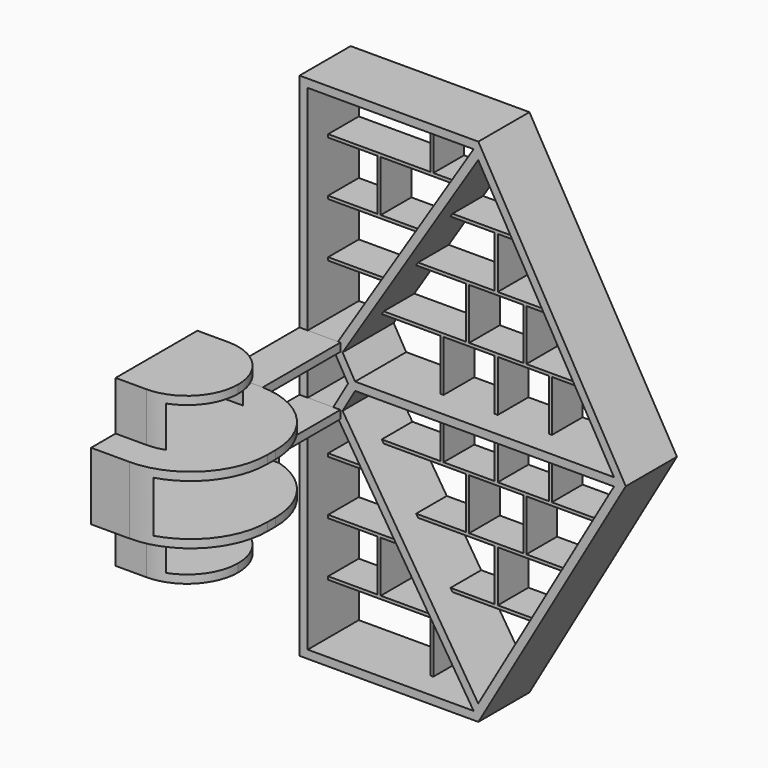
from build123d import *

# Parameters (mm, degrees)
F2_DEPTH    = 125
F1_W        = 6
F1_H        = 100
F3_DEPTH    = 75
F4_W        = 6
F4_H        = 80
F5_DEPTH    = 160
F4_H_2      = 100
F6_DEPTH    = 80
F7_R        = 99.99999
F7_2_R      = 99.99999
F8_DEPTH    = 225
F9_T1_DEPTH = 882


# Not quite as in the source:
# - a fillet or chamfer that OpenCascade refuses, or shapes differently, is made with other operations: its cross-section is extruded or revolved along the edge and cut away or added
# - a fillet or chamfer is up to 0.001 mm smaller than in the source, because OpenCascade refuses the exact size
# - a feature names something its author has since deleted; it is built from what else it names


with BuildPart() as f2:
    # F1 (on Front) → F2 (new body)
    with BuildSketch(Plane.XZ):
        Polygon((0, 1000), (0, 0), (350, 0), (638.6751345948, 500), (350, 1000), align=None)
        Polygon((16, 884), (16, 984), (216, 984), (222, 984), (340.762395693, 984), (349.7876249334, 968.3678444056), (431.9837382249, 826), (435.4478398401, 820), (493.182866759, 720), (496.6469683742, 714), (554.3819952931, 614), (557.8460969083, 608), (615.5811238272, 508), (620.1999259807, 500), (615.5811238272, 492), (557.8460969083, 392), (554.3819952931, 386), (496.6469683742, 286), (493.182866759, 280), (435.4478398401, 180), (431.9837382249, 174), (349.7876249334, 31.6321555944), (340.762395693, 16), (222, 16), (216, 16), (16, 16), (16, 116), (16, 122), (16, 222), (16, 228), (16, 328), (16, 334), (16, 434), (16, 450), (16, 550), (16, 566), (16, 666), (16, 672), (16, 772), (16, 778), (16, 878), align=None, mode=Mode.SUBTRACT)
        Polygon((236.0177204531, 508), (108.72391992, 508), (113.3427220735, 500), (108.72391992, 492), (236.0177204531, 492), (242.0177204531, 492), (342.0177204531, 492), (348.0177204531, 492), (448.0177204531, 492), (454.0177204531, 492), (615.5811238272, 492), (620.1999259807, 500), (615.5811238272, 508), (454.0177204531, 508), (448.0177204531, 508), (348.0177204531, 508), (342.0177204531, 508), (242.0177204531, 508), align=None)
        Polygon((84.2628335475, 449.6321555944), (75.237604307, 434), (138.7602816721, 334), (142.571642314, 328), (206.094319679, 228), (209.905680321, 222), (273.428357686, 122), (277.2397183279, 116), (340.762395693, 16), (349.7876249334, 31.6321555944), (259.3517584601, 174), (255.5403978182, 180), (192.0177204531, 280), (188.2063598112, 286), (124.6836824461, 386), (120.8723218042, 392), align=None)
        Polygon((349.7876249334, 968.3678444056), (340.762395693, 984), (277.2397183279, 884), (273.428357686, 878), (209.905680321, 778), (206.094319679, 772), (142.571642314, 672), (138.7602816721, 666), (75.237604307, 566), (84.2628335475, 550.3678444056), (120.8723218042, 608), (124.6836824461, 614), (188.2063598112, 714), (192.0177204531, 720), (255.5403978182, 820), (259.3517584601, 826), align=None)
        Polygon((75.237604307, 566), (16, 566), (16, 550), (66, 550), (94.8675134595, 500), (66, 450), (16, 450), (16, 434), (75.237604307, 434), (84.2628335475, 449.6321555944), (108.72391992, 492), (113.3427220735, 500), (108.72391992, 508), (84.2628335475, 550.3678444056), align=None)
    extrude(amount=F2_DEPTH)

    # F1 (on Front) → F3 (join)
    with BuildSketch(Plane.XZ):
        Polygon((112.9528401605, 122), (16, 122), (16, 116), (216, 116), (222, 116), (277.2397183279, 116), (273.428357686, 122), (118.9528401605, 122), align=None)
        with Locations((219, 66)):
            Rectangle(F1_W, F1_H)
        with Locations((115.9528401605, 172)):
            Rectangle(F1_W, F1_H)
        Polygon((206.094319679, 228), (16, 228), (16, 222), (112.9528401605, 222), (118.9528401605, 222), (209.905680321, 222), align=None)
        Polygon((138.7602816721, 334), (16, 334), (16, 328), (142.571642314, 328), align=None)
        Polygon((342.0177204531, 180), (255.5403978182, 180), (259.3517584601, 174), (431.9837382249, 174), (435.4478398401, 180), (348.0177204531, 180), align=None)
        with Locations((345.0177204531, 230)):
            Rectangle(F1_W, F1_H)
        Polygon((286.0177204531, 286), (188.2063598112, 286), (192.0177204531, 280), (342.0177204531, 280), (348.0177204531, 280), (493.182866759, 280), (496.6469683742, 286), (404.0177204531, 286), (398.0177204531, 286), (292.0177204531, 286), align=None)
        with Locations((289.0177204531, 336)):
            Rectangle(F1_W, F1_H)
        with Locations((401.0177204531, 336)):
            Rectangle(F1_W, F1_H)
        Polygon((236.0177204531, 392), (120.8723218042, 392), (124.6836824461, 386), (286.0177204531, 386), (292.0177204531, 386), (398.0177204531, 386), (404.0177204531, 386), (554.3819952931, 386), (557.8460969083, 392), (454.0177204531, 392), (448.0177204531, 392), (348.0177204531, 392), (342.0177204531, 392), (242.0177204531, 392), align=None)
        with Locations((345.0177204531, 442)):
            Rectangle(F1_W, F1_H)
        with Locations((239.0177204531, 442)):
            Rectangle(F1_W, F1_H)
        with Locations((451.0177204531, 442)):
            Rectangle(F1_W, F1_H)
        with Locations((401.0177204531, 664)):
            Rectangle(F1_W, F1_H)
        Polygon((496.6469683742, 714), (493.182866759, 720), (348.0177204531, 720), (342.0177204531, 720), (192.0177204531, 720), (188.2063598112, 714), (286.0177204531, 714), (292.0177204531, 714), (398.0177204531, 714), (404.0177204531, 714), align=None)
        with Locations((345.0177204531, 770)):
            Rectangle(F1_W, F1_H)
        Polygon((557.8460969083, 608), (554.3819952931, 614), (404.0177204531, 614), (398.0177204531, 614), (292.0177204531, 614), (286.0177204531, 614), (124.6836824461, 614), (120.8723218042, 608), (236.0177204531, 608), (242.0177204531, 608), (342.0177204531, 608), (348.0177204531, 608), (448.0177204531, 608), (454.0177204531, 608), align=None)
        with Locations((451.0177204531, 558)):
            Rectangle(F1_W, F1_H)
        with Locations((239.0177204531, 558)):
            Rectangle(F1_W, F1_H)
        with Locations((345.0177204531, 558)):
            Rectangle(F1_W, F1_H)
        Polygon((142.571642314, 672), (16, 672), (16, 666), (138.7602816721, 666), align=None)
        Polygon((112.9528401605, 778), (16, 778), (16, 772), (206.094319679, 772), (209.905680321, 778), (118.9528401605, 778), align=None)
        with Locations((115.9528401605, 828)):
            Rectangle(F1_W, F1_H)
        Polygon((216, 884), (16, 884), (16, 878), (112.9528401605, 878), (118.9528401605, 878), (273.428357686, 878), (277.2397183279, 884), (222, 884), align=None)
        with Locations((219, 934)):
            Rectangle(F1_W, F1_H)
        Polygon((435.4478398401, 820), (431.9837382249, 826), (259.3517584601, 826), (255.5403978182, 820), (342.0177204531, 820), (348.0177204531, 820), align=None)
        with Locations((289.0177204531, 664)):
            Rectangle(F1_W, F1_H)
    extrude(amount=F3_DEPTH)


with BuildPart() as f5:
    # F4 (on Right) → F5 (new body)
    with BuildSketch(Plane.YZ):
        Polygon((-381, 646), (-375, 646), (-375, 662), (-575, 662), (-575, 646), (-569, 646), align=None)
        with Locations((-572, 606)):
            Rectangle(F4_W, F4_H)
        with Locations((-378, 606)):
            Rectangle(F4_W, F4_H)
    extrude(amount=F5_DEPTH)

    # F7 (radius 100 in the source; OpenCascade refuses exactly that, so slightly less here)
    f7_edges = [f5.edges().sort_by_distance(p)[0] for p in [
        (160, -375, 614),
        (160, -575, 614),
    ]]
    fillet(f7_edges, radius=F7_R)


with BuildPart() as f5b:
    # F4 (on Right) → F5, piece 2 (new body)
    with BuildSketch(Plane.YZ):
        Polygon((-375, 338), (-375, 354), (-381, 354), (-569, 354), (-575, 354), (-575, 338), align=None)
        with Locations((-378, 394)):
            Rectangle(F4_W, F4_H)
        with Locations((-572, 394)):
            Rectangle(F4_W, F4_H)
    extrude(amount=F5_DEPTH)

    # F7#2 (radius 100 in the source; OpenCascade refuses exactly that, so slightly less here)
    f7_2_edges = [f5b.edges().sort_by_distance(p)[0] for p in [
        (160, -375, 386),
        (160, -575, 386),
    ]]
    fillet(f7_2_edges, radius=F7_2_R)


with BuildPart() as f6:
    # F4 (on Right) → F6 (new body)
    with BuildSketch(Plane.YZ):
        with Locations((-312, 500)):
            Rectangle(F4_W, F4_H_2)
        Polygon((-309, 550), (-125, 550), (-125, 566), (-315, 566), (-315, 550), align=None)
        Polygon((-125, 450), (-309, 450), (-315, 450), (-315, 434), (-125, 434), align=None)
    extrude(amount=F6_DEPTH)


with BuildPart() as f8:
    # F4 (on Right) → F8 (new body)
    with BuildSketch(Plane.YZ):
        Polygon((-321, 550), (-315, 550), (-315, 566), (-375, 566), (-381, 566), (-569, 566), (-575, 566), (-635, 566), (-635, 550), (-629, 550), align=None)
        with Locations((-632, 500)):
            Rectangle(F4_W, F4_H_2)
        Polygon((-315, 434), (-315, 450), (-321, 450), (-629, 450), (-635, 450), (-635, 434), (-575, 434), (-569, 434), (-381, 434), (-375, 434), align=None)
        with Locations((-318, 500)):
            Rectangle(F4_W, F4_H_2)
    extrude(amount=F8_DEPTH)

    # F9: fillet of radius 150 on 2 edges, made by hand

    # F9_s2 → F9_t1 (cut)
    with BuildSketch(Plane.XY.offset(59)):
        with BuildLine():
            ThreePointArc((75, -635), (181.066017178, -591.066017178), (225, -485))
            Line((225, -485), (225, -635))
            Line((225, -635), (75, -635))
        make_face()
        with BuildLine():
            ThreePointArc((75, -315), (181.066017178, -358.933982822), (225, -465))
            Line((225, -465), (225, -315))
            Line((225, -315), (75, -315))
        make_face()
    extrude(amount=F9_T1_DEPTH, mode=Mode.SUBTRACT)


solid = Compound([f2.part, f5.part, f5b.part, f6.part, f8.part])
